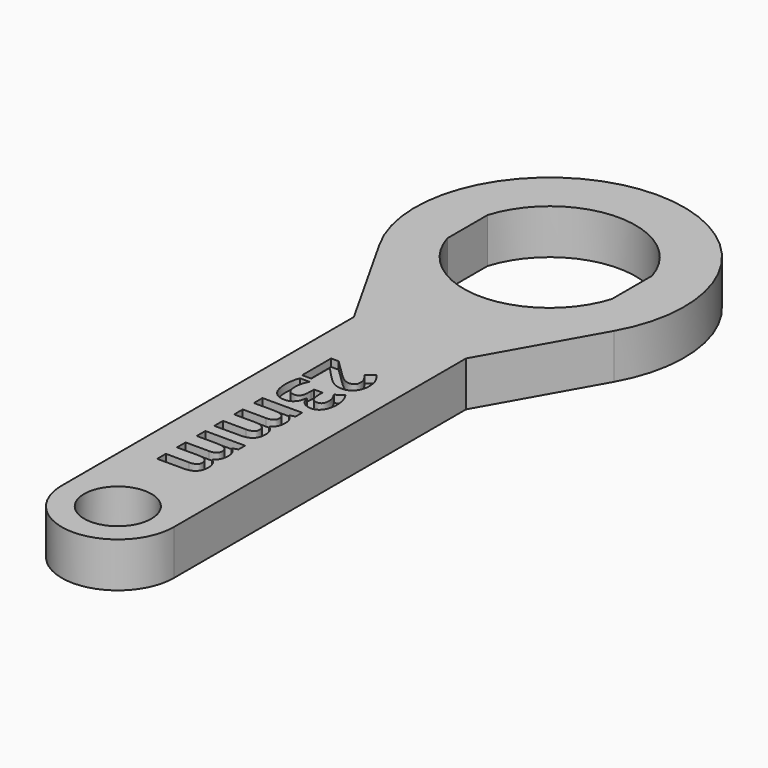
from build123d import *

# Parameters (mm, degrees)
F0_R         = 4.5
F1_DEPTH     = 6
F2_TEXT_SIZE = 9.7222222222
F3_DEPTH     = 1


# Not quite as in the source:
# - Text() gives the source's letters only with a copy of the font that has no kerning and outlines rounded to 1/6400 em; it was checked with that copy


with BuildPart() as f1:
    # F0 (on Top) → F1 (new body)
    with BuildSketch(Plane.XY):
        with BuildLine():
            Line((7.5, -23.363068172), (15.6835024996, -8.833331724))
            ThreePointArc((15.6835024996, -8.833331724), (0, 18), (-15.6835024996, -8.833331724))
            Line((-15.6835024996, -8.833331724), (-7.5, -23.363068172))
            Line((-7.5, -23.363068172), (-7.5, -72.1933111548))
            ThreePointArc((-7.5, -72.1933111548), (-5.3033008589, -77.4966120137), (0, -79.6933111548))
            ThreePointArc((0, -79.6933111548), (5.3033008589, -77.4966120137), (7.5, -72.1933111548))
            Line((7.5, -72.1933111548), (7.5, -23.363068172))
        make_face()
        with Locations((0, -72.1933111548)):
            Circle(F0_R, mode=Mode.SUBTRACT)
        with BuildLine():
            ThreePointArc((11, -3.3541019662), (0, -11.5), (-11, -3.3541019662))
            Line((-11, -3.3541019662), (-11, 3.3541019662))
            ThreePointArc((-11, 3.3541019662), (0, 11.5), (11, 3.3541019662))
            Line((11, 3.3541019662), (11, -3.3541019662))
        make_face(mode=Mode.SUBTRACT)
    extrude(amount=F1_DEPTH)

    # F2 (on face) → F3 (cut)
    with BuildSketch(Plane.XY.offset(6)):
        with Locations(Location((-3.5, -31.7741170989), (0, 0, -90))):
            Text('23mm', F2_TEXT_SIZE, font='Open Sans', font_style=FontStyle.BOLD, text_align=(TextAlign.LEFT, TextAlign.BOTTOM))
    extrude(amount=-F3_DEPTH, mode=Mode.SUBTRACT)


solid = f1.part
